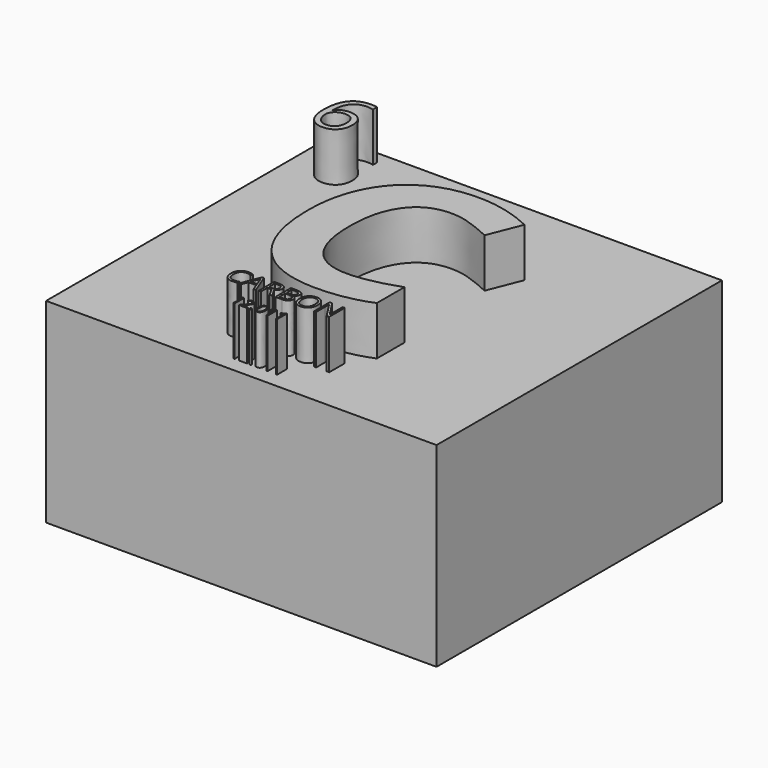
from build123d import *

# Parameters (mm, degrees)
F0_W           = 20
F0_H           = 18.2727293761
F1_DEPTH       = 10
F2_TEXT_SIZE   = 13.8888888889
F2_TEXT_SIZE_2 = 3.7478047708
F1_FACE1_W     = 20
F1_FACE1_H     = 18.2727293761
F3_DEPTH       = 2.5
F4_TEXT_SIZE   = 1.3888888889
F4_TEXT_SIZE_2 = 0.8547005463
F5_DEPTH       = 2.5


# Not quite as in the source:
# - Text() gives the source's letters only with a copy of the font that has no kerning and outlines rounded to 1/6400 em; it was checked with that copy


with BuildPart() as f1:
    # F0 (on Top) → F1 (new body)
    with BuildSketch(Plane.XY):
        Rectangle(F0_W, F0_H)
    extrude(amount=F1_DEPTH)

    # F2 (on face) + F1_face1 (on face) → F3 (join)
    with BuildSketch(Plane.XY.offset(10)):
        with Locations((-4.5383128687, -5.1440539276)):
            Text('C', F2_TEXT_SIZE, font='Open Sans', font_style=FontStyle.BOLD, text_align=(TextAlign.LEFT, TextAlign.BOTTOM))
        with Locations((-8.9016797961, 5.8056821072)):
            Text('6', F2_TEXT_SIZE_2, font='Open Sans', text_align=(TextAlign.LEFT, TextAlign.BOTTOM))
    with BuildSketch(Plane(origin=(0, 0, 0), x_dir=(1, 0, 0), z_dir=(0, 0, -1))):
        Rectangle(F1_FACE1_W, F1_FACE1_H)
    extrude(amount=F3_DEPTH, dir=(0, 0, 1))

    # F4 (on face) → F5 (join)
    with BuildSketch(Plane.XY.offset(10)):
        with Locations((-2.7980685764, -6.8914601515)):
            Text('CARBON', F4_TEXT_SIZE, font='Open Sans', text_align=(TextAlign.LEFT, TextAlign.BOTTOM))
        with Locations((-1.2678948416, -8.3509039821)):
            Text('12.011', F4_TEXT_SIZE_2, font='Open Sans', text_align=(TextAlign.LEFT, TextAlign.BOTTOM))
    extrude(amount=F5_DEPTH)


solid = f1.part
